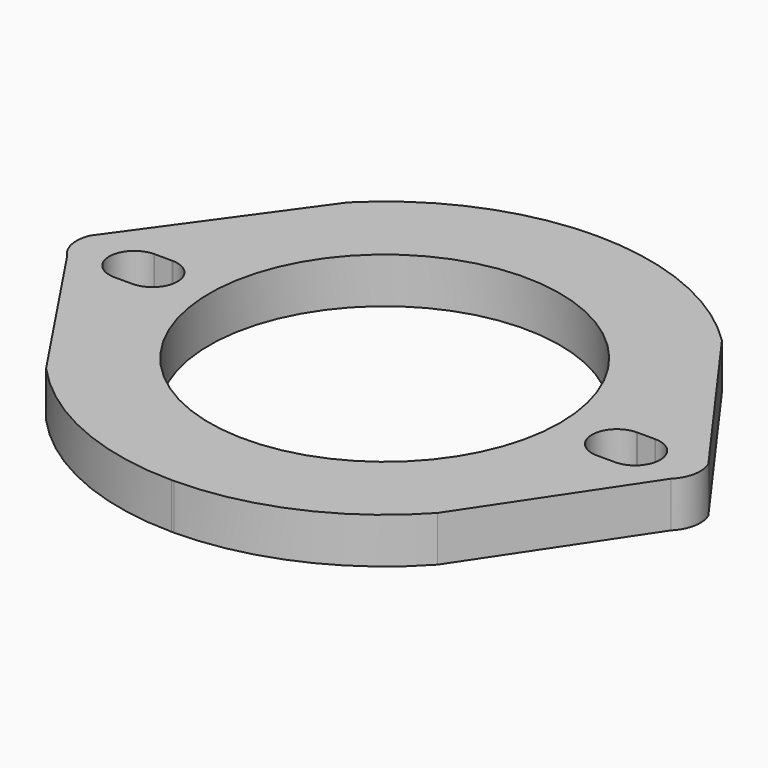
from build123d import *

# Parameters (mm, degrees)
F0_R     = 38.5
F1_DEPTH = 10


# Not quite as in the source:
# - a feature names something its author has since deleted; it is built from what else it names


with BuildPart() as f1:
    # F0 (on Top) → F1 (new body)
    with BuildSketch(Plane.XY):
        with BuildLine():
            Line((-66.2866235273, -4.2965270375), (-42.9791214207, -39.2359080502))
            ThreePointArc((-42.9791214207, -39.2359080502), (-23.5911513271, -53.1988621842), (-0.226643991, -58.1945873009))
            ThreePointArc((-0.226643991, -58.1945873009), (0, -58.1950286418), (0.226643991, -58.1945873009))
            ThreePointArc((0.226643991, -58.1945873009), (23.5911513271, -53.1988621842), (42.9791214207, -39.2359080502))
            Line((42.9791214207, -39.2359080502), (66.2866235273, -4.2965270375))
            ThreePointArc((66.2866235273, -4.2965270375), (68.3602831702, -0.4175146073), (67.9024238921, 3.9570901325))
            Line((67.9024238921, 3.9570901325), (65.9713692122, 6.6390455982))
            Line((65.9713692122, 6.6390455982), (41.053212855, 41.2467583321))
            ThreePointArc((41.053212855, 41.2467583321), (22.3169041562, 53.7458570265), (0.2378206695, 58.1945426991))
            ThreePointArc((0.2378206695, 58.1945426991), (0, 58.1950286418), (-0.2378206695, 58.1945426991))
            ThreePointArc((-0.2378206695, 58.1945426991), (-22.3169041562, 53.7458570265), (-41.053212855, 41.2467583321))
            Line((-41.053212855, 41.2467583321), (-65.9713692122, 6.6390455982))
            Line((-65.9713692122, 6.6390455982), (-67.9024238921, 3.9570901325))
            ThreePointArc((-67.9024238921, 3.9570901325), (-68.3602831702, -0.4175146073), (-66.2866235273, -4.2965270375))
        make_face()
        with BuildLine():
            ThreePointArc((-55.0301875187, 5.4990596786), (-54.9860185236, 5.499237036), (-54.9418495285, 5.4990596786))
            Line((-54.9418495285, 5.4990596786), (-51.1476298855, 5.4990596786))
            ThreePointArc((-51.1476298855, 5.4990596786), (-51.013562259, 5.500693933), (-50.8794946326, 5.4990596786))
            ThreePointArc((-50.8794946326, 5.4990596786), (-45.5139634735, -0.065737976), (-51.0123484011, -5.499305933))
            Line((-51.0123484011, -5.499305933), (-54.9049202804, -5.5001650292))
            ThreePointArc((-54.9049202804, -5.5001650292), (-60.4856618743, -0.0633969362), (-55.0301875187, 5.4990596786))
        make_face(mode=Mode.SUBTRACT)
        Circle(F0_R, mode=Mode.SUBTRACT)
        with BuildLine():
            ThreePointArc((55.0301875187, 5.4990596786), (60.4856618743, -0.0633969362), (54.9049202804, -5.5001650292))
            Line((54.9049202804, -5.5001650292), (51.0123484011, -5.499305933))
            ThreePointArc((51.0123484011, -5.499305933), (45.5139634735, -0.065737976), (50.8794946326, 5.4990596786))
            ThreePointArc((50.8794946326, 5.4990596786), (51.013562259, 5.500693933), (51.1476298855, 5.4990596786))
            Line((51.1476298855, 5.4990596786), (54.9418495285, 5.4990596786))
            ThreePointArc((54.9418495285, 5.4990596786), (54.9860185236, 5.499237036), (55.0301875187, 5.4990596786))
        make_face(mode=Mode.SUBTRACT)
    extrude(amount=-F1_DEPTH)


solid = f1.part
